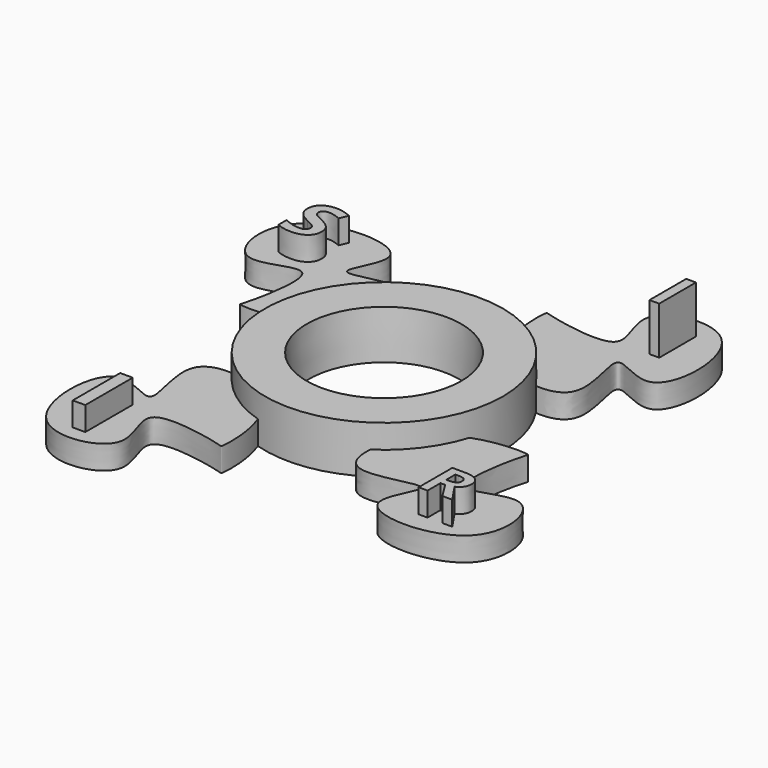
from build123d import *

# Parameters (mm, degrees)
F0_R          = 17.5
F1_DEPTH      = 7
F2_R          = 11
F3_DEPTH      = 25
F3_TAPER      = -3
F5_DEPTH      = 3.5
F6_COUNT      = 4
F7_TEXT_SIZE  = 9.4594589124
F8_DEPTH      = 7
F9_TEXT_SIZE  = 8.6711719632
F10_DEPTH     = 7
F11_TEXT_SIZE = 12.2184684086
F12_DEPTH     = 7
F13_TEXT_SIZE = 10.6418919232
F14_DEPTH     = 7


# Not quite as in the source:
# - Text() gives the source's letters only with a copy of the font that has no kerning and outlines rounded to 1/6400 em; it was checked with that copy


with BuildPart() as f1:
    # F0 (on Top) → F1 (new body)
    with BuildSketch(Plane.XY):
        Circle(F0_R)
    extrude(amount=F1_DEPTH)

    # F2 (on Top) → F3 (cut)
    with BuildSketch(Plane.XY):
        Circle(F2_R)
    extrude(amount=F3_DEPTH, taper=F3_TAPER, mode=Mode.SUBTRACT)

    # F4 (on Top) → F5 (join)
    with BuildSketch(Plane.XY):
        with BuildLine():
            add(Edge.make_bspline(
                [(6.8201594986, 13.7655679137), (3.6845637607, 17.6522178762), (4.0687578065, 24.86098991), (4.4900692102, 24.4350955384), (19.5513020375, 20.825233503), (9.9898989191, 32.9789240933), (27.6917524819, 36.2829658498), (27.2703784451, 13.792836503), (15.1314006584, 24.1047226946), (23.3179612256, 7.0378891554), (10.1134156344, 9.6834939135), (6.8201594986, 13.7655679137)],
                knots=[0, 0, 0, 0, 0.1304890466, 0.1494630233, 0.2754679204, 0.3813568258, 0.5045999174, 0.647894104, 0.7459057177, 0.8629498541, 1, 1, 1, 1], degree=3))
        make_face()
    extrude(amount=F5_DEPTH)

    # F6: F1 ×4 about axis
    f6_axis = Axis((0, 0, 7), (0, 0, 1))


with BuildPart() as f1_1:
    add(f1.part)
    for i in range(1, F6_COUNT):
        add(f1.part.rotate(f6_axis, i * 360 / F6_COUNT))

    # F7 (on face) → F8 (join)
    with BuildSketch(Plane.XY.offset(3.5)):
        with Locations((19.0135091543, 23.9797290415)):
            Text('I', F7_TEXT_SIZE, font='Open Sans', font_style=FontStyle.BOLD, text_align=(TextAlign.LEFT, TextAlign.BOTTOM))
    extrude(amount=F8_DEPTH)

    # F9 (on Top) → F10 (join)
    with BuildSketch(Plane.XY):
        with Locations((23.2702698559, -23.6959476024)):
            Text('R', F9_TEXT_SIZE, font='Open Sans', font_style=FontStyle.BOLD, text_align=(TextAlign.LEFT, TextAlign.BOTTOM))
    extrude(amount=F10_DEPTH)

    # F11 (on Top) → F12 (join)
    with BuildSketch(Plane.XY):
        with Locations((-21.5675681829, -31.6418930888)):
            Text('I', F11_TEXT_SIZE, font='Open Sans', font_style=FontStyle.BOLD, text_align=(TextAlign.LEFT, TextAlign.BOTTOM))
    extrude(amount=F12_DEPTH)

    # F13 (on Top) → F14 (join)
    with BuildSketch(Plane.XY):
        with Locations((-29.7972988337, 16.8851353228)):
            Text('S', F13_TEXT_SIZE, font='Open Sans', font_style=FontStyle.BOLD, text_align=(TextAlign.LEFT, TextAlign.BOTTOM))
    extrude(amount=F14_DEPTH)


solid = f1_1.part
